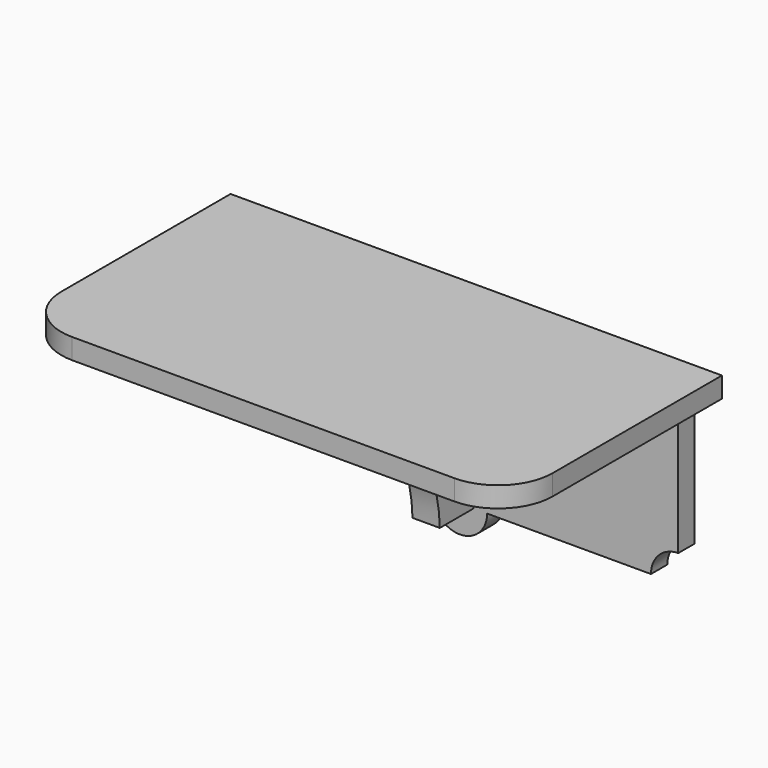
from build123d import *

# Parameters (mm, degrees)
F1_DEPTH  = 9.525
F2_W      = 12.7
F2_H      = 9.525
F2_W_2    = 203.2
F3_DEPTH  = 9.525
F5_DEPTH  = 114.3
F7_DEPTH  = 9.652
F8_DEPTH  = 25.4
F9_W      = 12.7
F9_H      = 76.2
F10_DEPTH = 88.9
F12_DEPTH = 25.4


with BuildPart() as f1:
    # F0 (on Front) → F1 (new body)
    with BuildSketch(Plane.XZ):
        with BuildLine():
            Line((100.1874667764, 17.9892315423), (-103.0125332236, 17.9892315423))
            Line((-103.0125332236, 17.9892315423), (-103.0125332236, -45.5107684577))
            ThreePointArc((-103.0125332236, -45.5107684577), (-94.0322771026, -49.2305123366), (-90.3125332236, -58.2107684577))
            Line((-90.3125332236, -58.2107684577), (-14.1125332236, -58.2107684577))
            ThreePointArc((-14.1125332236, -58.2107684577), (-1.4125332236, -70.9107684577), (11.2874667764, -58.2107684577))
            Line((11.2874667764, -58.2107684577), (87.4874667764, -58.2107684577))
            ThreePointArc((87.4874667764, -58.2107684577), (91.2072106553, -49.2305123366), (100.1874667764, -45.5107684577))
            Line((100.1874667764, -45.5107684577), (100.1874667764, 17.9892315423))
        make_face()
    extrude(amount=F1_DEPTH)

    # F2 (on face) → F3 (join)
    with BuildSketch(Plane.XY.offset(17.9892315423)):
        with Locations((-109.3625332236, -4.7625)):
            Rectangle(F2_W, F2_H)
        with Locations((-1.4125332236, -4.7625)):
            Rectangle(F2_W_2, F2_H)
        with Locations((106.5374667764, -4.7625)):
            Rectangle(F2_W, F2_H)
    extrude(amount=F3_DEPTH)

    # F4 (on face) → F5 (join)
    with BuildSketch(Plane.XZ.offset(9.525)):
        Polygon((-115.7125332236, 17.9892315423), (-103.0125332236, 17.9892315423), (100.1874667764, 17.9892315423), (112.8874667764, 17.9892315423), (112.8874667764, 27.5142315423), (-115.7125332236, 27.5142315423), align=None)
    extrude(amount=F5_DEPTH)

    # F6 (on face) → F7 (cut)
    with BuildSketch(Plane.XY.offset(27.5142315423)):
        with BuildLine():
            ThreePointArc((-90.3125332236, -123.825), (-108.2730454658, -116.3855122421), (-115.7125332236, -98.425))
            Line((-115.7125332236, -98.425), (-115.7125332236, -123.825))
            Line((-115.7125332236, -123.825), (-90.3125332236, -123.825))
        make_face()
    extrude(amount=-F7_DEPTH, mode=Mode.SUBTRACT)

    # F6 (on face) → F8 (cut)
    with BuildSketch(Plane.XY.offset(27.5142315423)):
        with BuildLine():
            Line((112.8874667764, -123.825), (112.8874667764, -98.425))
            ThreePointArc((112.8874667764, -98.425), (105.4479790185, -116.3855122421), (87.4874667764, -123.825))
            Line((87.4874667764, -123.825), (112.8874667764, -123.825))
        make_face()
    extrude(amount=-F8_DEPTH, mode=Mode.SUBTRACT)

    # F9 (on face) → F10 (join)
    with BuildSketch(Plane.XZ.offset(9.525)):
        with Locations((-1.4125332236, -20.1107684577)):
            Rectangle(F9_W, F9_H)
    extrude(amount=F10_DEPTH)

    # F11 (on face) → F12 (cut)
    with BuildSketch(Plane.YZ.offset(4.9374667764)):
        with BuildLine():
            ThreePointArc((-29.1272475292, -58.2107684577), (-50.2201883101, -11.5676739355), (-98.425, 5.659820001))
            Line((-98.425, 5.659820001), (-98.425, 5.2892315423))
            Line((-98.425, 5.2892315423), (-98.425, -58.2107684577))
            Line((-98.425, -58.2107684577), (-29.1272475292, -58.2107684577))
        make_face()
    extrude(amount=-F12_DEPTH, mode=Mode.SUBTRACT)


solid = f1.part
